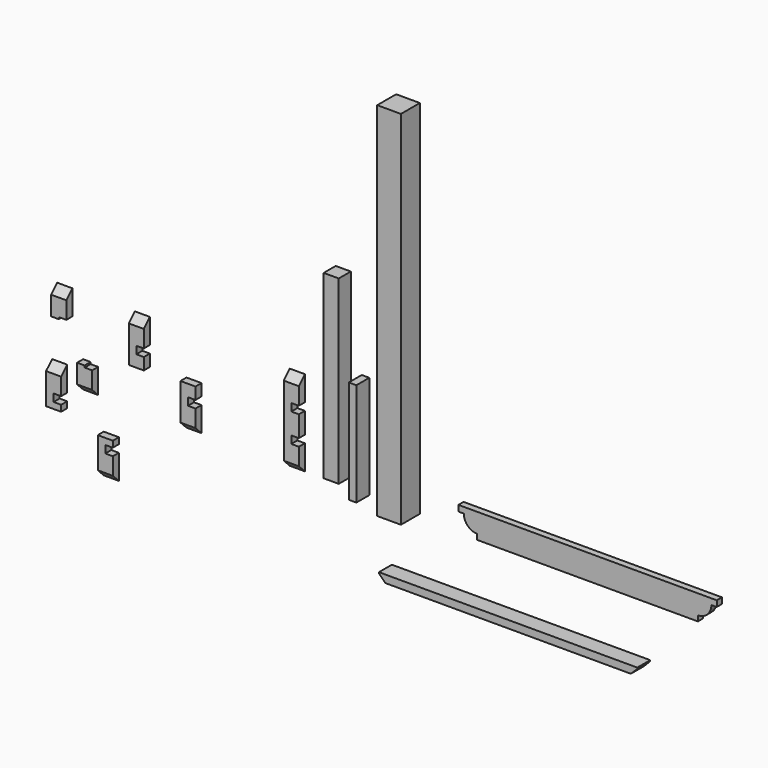
from build123d import *

# Parameters (mm, degrees)
F0_W      = 139.7
F0_H      = 2133.6
F1_DEPTH  = 139.7
F3_DEPTH  = 38.1
F5_DEPTH  = 95.25
F6_W      = 88.9
F6_H      = 88.9
F7_DEPTH  = 1066.8
F8_W      = 44.45
F8_H      = 609.6
F9_DEPTH  = 95.25
F11_DEPTH = 44.45
F13_DEPTH = 88.9
F16_DEPTH = 101.6
F18_W     = 44.45
F18_H     = 242.5570257008
F18_H_2   = 53.975
F19_DEPTH = 101.6
F21_W     = 44.45
F21_H     = 190.5
F21_H_2   = 123.825
F21_H_3   = 33.3248
F22_DEPTH = 101.6
F24_W     = 44.45
F24_H     = 123.825
F25_DEPTH = 101.6
F27_W     = 44.45
F27_H     = 87.3252
F27_H_2   = 192.8097355843
F28_DEPTH = 101.6
F30_W     = 44.45
F30_H     = 87.3252
F31_DEPTH = 101.6


with BuildPart() as f1:
    # F0 (on Front) → F1 (new body)
    with BuildSketch(Plane.XZ):
        with Locations((95.25, 1066.8)):
            Rectangle(F0_W, F0_H)
    extrude(amount=F1_DEPTH)


with BuildPart() as f3:
    # F2 (on Front) → F3 (new body)
    with BuildSketch(Plane.XZ):
        with BuildLine():
            Line((534.11054703, 31.75), (534.11054703, 0))
            Line((534.11054703, 0), (1835.86054703, 0))
            Line((1835.86054703, 0), (1835.86054703, 31.75))
            ThreePointArc((1835.86054703, 31.75), (1891.9871477866, 54.9983992433), (1915.23554703, 111.125))
            Line((1915.23554703, 111.125), (1946.98554703, 111.125))
            Line((1946.98554703, 111.125), (1946.98554703, 146.05))
            Line((1946.98554703, 146.05), (422.98554703, 146.05))
            Line((422.98554703, 146.05), (422.98554703, 111.125))
            Line((422.98554703, 111.125), (454.73554703, 111.125))
            ThreePointArc((454.73554703, 111.125), (477.9839462733, 54.9983992433), (534.11054703, 31.75))
        make_face()
    extrude(amount=F3_DEPTH)


with BuildPart() as f5:
    # F4 (on Front) → F5 (new body)
    with BuildSketch(Plane.XZ):
        Polygon((1524, -317.7578675234), (0, -317.7578675234), (0, -324.1078675234), (38.1, -362.2078675234), (1485.9, -362.2078675234), (1524, -324.1078675234), align=None)
    extrude(amount=F5_DEPTH)


with BuildPart() as f7:
    # F6 (on Top) → F7 (new body)
    with BuildSketch(Plane.XY):
        with Locations((-357.7766300052, 44.45)):
            Rectangle(F6_W, F6_H)
    extrude(amount=F7_DEPTH)


with BuildPart() as f9:
    # F8 (on Front) → F9 (new body)
    with BuildSketch(Plane.XZ):
        with Locations((-155.4375765641, 304.8)):
            Rectangle(F8_W, F8_H)
    extrude(amount=F9_DEPTH)


with BuildPart() as f11:
    # F10 (on Front) → F11 (new body)
    with BuildSketch(Plane.XZ):
        Polygon((-602.0738712236, 504.825), (-602.0738712236, 0), (-513.1738712236, 0), (-513.1738712236, 146.05), (-557.6238712236, 146.05), (-557.6238712236, 190.5), (-513.1738712236, 190.5), (-513.1738712236, 314.325), (-557.6238712236, 314.325), (-557.6238712236, 358.775), (-513.1738712236, 358.775), (-513.1738712236, 504.825), align=None)
    extrude(amount=F11_DEPTH)

    # F12 (on face) → F13 (cut)
    with BuildSketch(Plane(origin=(-602.0738712236, 0, 0), x_dir=(0, -1, 0), z_dir=(-1, 0, 0))):
        Polygon((44.45, 504.825), (0, 504.825), (44.45, 460.375), align=None)
        Polygon((44.45, 44.45), (0, 0), (44.45, 0), align=None)
    extrude(amount=-F13_DEPTH, mode=Mode.SUBTRACT)


with BuildPart() as f14_1:
    # F14: copy of F11
    add(f11.part.moved(Location((-609.6, 0, 0))))

    # F15 (on face) → F16 (cut)
    with BuildSketch(Plane.YZ.offset(-1122.7738712236)):
        Polygon((-45.72, 260.35), (0, 260.35), (0, 358.775), (-44.45, 358.775), (-44.45, 460.375), (0, 504.825), (0, 768.35), (-45.72, 768.35), align=None)
        Polygon((-44.45, 358.775), (0, 358.775), (0, 504.825), (-44.45, 460.375), align=None)
    extrude(amount=-F16_DEPTH, mode=Mode.SUBTRACT)


with BuildPart() as f17_1:
    # F17: copy of F11
    add(f11.part.moved(Location((-914.4, 0, 0))))

    # F18 (on face) → F19 (cut)
    with BuildSketch(Plane.YZ.offset(-1427.5738712236)):
        with Locations((-22.225, 69.2214871496)):
            Rectangle(F18_W, F18_H)
        with Locations((-22.225, 217.4875)):
            Rectangle(F18_W, F18_H_2)
    extrude(amount=-F19_DEPTH, mode=Mode.SUBTRACT)


with BuildPart() as f20_1:
    # F20: copy of F11
    add(f11.part.moved(Location((-1219.2, 0, 0))))

    # F21 (on face) → F22 (cut)
    with BuildSketch(Plane.YZ.offset(-1732.3738712236)):
        with Locations((-22.225, 409.575)):
            Rectangle(F21_W, F21_H)
        with Locations((-22.225, 252.4125)):
            Rectangle(F21_W, F21_H_2)
        with Locations((-22.225, 173.8376)):
            Rectangle(F21_W, F21_H_3)
    extrude(amount=-F22_DEPTH, mode=Mode.SUBTRACT)


with BuildPart() as f23_1:
    # F23: copy of F11
    add(f11.part.moved(Location((-1371.6, 0, 0))))

    # F24 (on face) → F25 (cut)
    with BuildSketch(Plane.YZ.offset(-1884.7738712236)):
        Polygon((-51.1882424594, 0), (0, 0), (0, 190.5), (-44.45, 190.5), (-44.45, 314.325), (0, 314.325), (0, 347.6498), (-51.1882424594, 347.6498), align=None)
        with Locations((-22.225, 252.4125)):
            Rectangle(F24_W, F24_H)
    extrude(amount=-F25_DEPTH, mode=Mode.SUBTRACT)


with BuildPart() as f26_1:
    # F26: copy of F11
    add(f11.part.moved(Location((-609.6, -609.6, 0))))

    # F27 (on face) → F28 (cut)
    with BuildSketch(Plane.YZ.offset(-1122.7738712236)):
        with Locations((-631.825, 270.6624)):
            Rectangle(F27_W, F27_H)
        with Locations((-631.825, 410.7298677921)):
            Rectangle(F27_W, F27_H_2)
    extrude(amount=-F28_DEPTH, mode=Mode.SUBTRACT)


with BuildPart() as f29_1:
    # F29: copy of F11
    add(f11.part.moved(Location((-914.4, -609.6, 0))))

    # F30 (on face) → F31 (cut)
    with BuildSketch(Plane.YZ.offset(-1427.5738712236)):
        Polygon((-654.05, 0), (-609.5743775368, 0), (-609.5743775368, 277.8252), (-609.6, 277.8252), (-609.6, 190.5), (-654.05, 190.5), align=None)
        with Locations((-631.825, 234.1626)):
            Rectangle(F30_W, F30_H)
    extrude(amount=-F31_DEPTH, mode=Mode.SUBTRACT)


solid = Compound([f1.part, f3.part, f5.part, f7.part, f9.part, f11.part, f14_1.part, f17_1.part, f20_1.part, f23_1.part, f26_1.part, f29_1.part])
